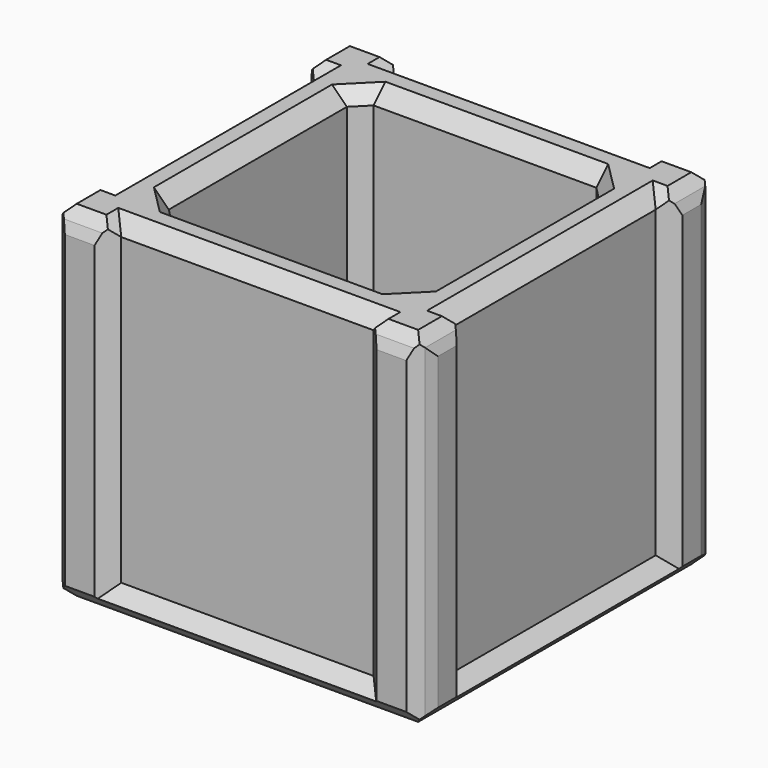
from build123d import *

# Parameters (mm, degrees)
F0_W          = 127
F0_H          = 127
F1_DEPTH      = 8.89
F2_W          = 86.36
F2_H          = 10.16
F2_W_2        = 10.16
F2_H_2        = 86.36
F3_DEPTH      = 101.6
F4_W          = 10.0171214116
F4_H          = 10.0171214116
F4_W_2        = 96.3771214116
F4_H_2        = 96.3771214116
F4_W_3        = 86.36
F4_H_3        = 86.36
F5_DEPTH      = 7.62
F6_W          = 86.36
F6_H          = 5.08
F9_W          = 5.08
F9_H          = 86.36
F7_W          = 5.08
F7_H          = 86.36
F8_W          = 86.36
F8_H          = 5.08
F10_DEPTH     = 109.22
F11_SIZE      = 5.08
F12_T1_DEPTH  = 139.1582991577
F12_T3_DEPTH  = 31.7862799398
F12_T5_DEPTH  = 153.1282991577
F12_T7_DEPTH  = 117.2041495789
F12_T9_DEPTH  = 86.36
F12_T11_DEPTH = 31.7862799398
F12_T17_DEPTH = 130.2682991577
F12_T22_DEPTH = 99.4241495789
F12_T29_DEPTH = 99.4241495789
F12_T33_DEPTH = 130.2682991577
F12_T41_DEPTH = 130.2682991577
F12_T46_DEPTH = 99.4241495789
F12_T53_DEPTH = 99.4241495789
F12_T57_DEPTH = 130.2682991577
F13_T1_DEPTH  = 124.4962799399
F13_T3_DEPTH  = 142.9682991577
F13_T5_DEPTH  = 26.7062799397
F13_T7_DEPTH  = 117.2041495789
F13_T9_DEPTH  = 86.36
F13_T11_DEPTH = 26.7062799398
F13_T17_DEPTH = 130.2682991577
F13_T22_DEPTH = 99.4241495789
F13_T29_DEPTH = 99.4241495789
F13_T33_DEPTH = 130.2682991577
F13_T41_DEPTH = 130.2682991577
F13_T46_DEPTH = 99.4241495789
F13_T53_DEPTH = 99.4241495789
F13_T57_DEPTH = 130.2682991577


# Not quite as in the source:
# - a fillet or chamfer that OpenCascade refuses, or shapes differently, is made with other operations: its cross-section is extruded or revolved along the edge and cut away or added


with BuildPart() as f1:
    # F0 (on Top) → F1 (new body)
    with BuildSketch(Plane.XY):
        with Locations((3.7135761231, -7.4630701935)):
            Rectangle(F0_W, F0_H)
    extrude(amount=F1_DEPTH)

    # F2 (on face) → F3 (join)
    with BuildSketch(Plane.XY.offset(8.89)):
        Polygon((-59.7864238769, 56.0369298065), (-59.7864238769, 35.7169298065), (-49.6264238769, 35.7169298065), (-39.4664238769, 35.7169298065), (-39.4664238769, 45.8769298065), (-39.4664238769, 56.0369298065), align=None)
        with Locations((3.7135761231, 40.7969298065)):
            Rectangle(F2_W, F2_H)
        Polygon((46.8935761231, 45.8769298065), (46.8935761231, 35.7169298065), (57.0535761231, 35.7169298065), (67.2135761231, 35.7169298065), (67.2135761231, 56.0369298065), (46.8935761231, 56.0369298065), align=None)
        with Locations((51.9735761231, -7.4630701935)):
            Rectangle(F2_W_2, F2_H_2)
        with Locations((-44.5464238769, -7.4630701935)):
            Rectangle(F2_W_2, F2_H_2)
        Polygon((-59.7864238769, -50.6430701935), (-59.7864238769, -70.9630701935), (-39.4664238769, -70.9630701935), (-39.4664238769, -60.8030701935), (-39.4664238769, -50.6430701935), (-49.6264238769, -50.6430701935), align=None)
        Polygon((46.8935761231, -60.8030701935), (46.8935761231, -70.9630701935), (67.2135761231, -70.9630701935), (67.2135761231, -50.6430701935), (57.0535761231, -50.6430701935), (46.8935761231, -50.6430701935), align=None)
        with Locations((3.7135761231, -55.7230701935)):
            Rectangle(F2_W, F2_H)
    extrude(amount=F3_DEPTH)

    # F4 (on face) → F5 (join)
    with BuildSketch(Plane.XY.offset(110.49)):
        Polygon((-39.4664238769, 56.0369298065), (-59.7864238769, 56.0369298065), (-59.7864238769, 35.7169298065), (-49.6264238769, 35.7169298065), (-49.6264238769, -50.6430701935), (-59.7864238769, -50.6430701935), (-59.7864238769, -70.9630701935), (-39.4664238769, -70.9630701935), (-39.4664238769, -60.8030701935), (46.8935761231, -60.8030701935), (46.8935761231, -70.9630701935), (67.2135761231, -70.9630701935), (67.2135761231, -50.6430701935), (57.0535761231, -50.6430701935), (57.0535761231, 35.7169298065), (67.2135761231, 35.7169298065), (67.2135761231, 56.0369298065), (46.8935761231, 56.0369298065), (46.8935761231, 45.8769298065), (-39.4664238769, 45.8769298065), align=None)
        with Locations((-49.6264238769, -60.8030701935)):
            Rectangle(F4_W, F4_H, mode=Mode.SUBTRACT)
        with Locations((57.0535761231, -60.8030701935)):
            Rectangle(F4_W, F4_H, mode=Mode.SUBTRACT)
        with Locations((-49.6264238769, 45.8769298065)):
            Rectangle(F4_W, F4_H, mode=Mode.SUBTRACT)
        with Locations((3.7135761231, -7.4630701935)):
            Rectangle(F4_W_2, F4_H_2, mode=Mode.SUBTRACT)
        with Locations((57.0535761231, 45.8769298065)):
            Rectangle(F4_W, F4_H, mode=Mode.SUBTRACT)
        with Locations((3.7135761231, -7.4630701935)):
            Rectangle(F4_W_2, F4_H_2)
        with Locations((3.7135761231, -7.4630701935)):
            Rectangle(F4_W_3, F4_H_3, mode=Mode.SUBTRACT)
        with Locations((-49.6264238769, 45.8769298065)):
            Rectangle(F4_W, F4_H)
        with Locations((57.0535761231, 45.8769298065)):
            Rectangle(F4_W, F4_H)
        with Locations((-49.6264238769, -60.8030701935)):
            Rectangle(F4_W, F4_H)
        with Locations((57.0535761231, -60.8030701935)):
            Rectangle(F4_W, F4_H)
    extrude(amount=F5_DEPTH)

    # F6 (on face) + F9 (on face) + F7 (on face) + F8 (on face) → F10 (join)
    with BuildSketch(Plane.XY.offset(8.89)):
        with Locations((3.7135761231, 48.4169298065)):
            Rectangle(F6_W, F6_H)
    with BuildSketch(Plane.XY.offset(8.89)):
        with Locations((-52.1664238769, -7.4630701935)):
            Rectangle(F9_W, F9_H)
    with BuildSketch(Plane.XY.offset(8.89)):
        with Locations((59.5935761231, -7.4630701935)):
            Rectangle(F7_W, F7_H)
    with BuildSketch(Plane.XY.offset(8.89)):
        with Locations((3.7135761231, -63.3430701935)):
            Rectangle(F8_W, F8_H)
    extrude(amount=F10_DEPTH)

    # F11
    f11_edges = [f1.edges().sort_by_distance(p)[0] for p in [
        (3.713576, -50.64307, 118.11),
        (-39.466424, -7.46307, 118.11),
        (3.713576, 35.71693, 118.11),
        (46.893576, -7.46307, 118.11),
        (67.213576, 45.87693, 118.11),
        (57.053576, 56.03693, 118.11),
        (46.893576, 53.49693, 118.11),
        (3.713576, 50.95693, 118.11),
        (-39.466424, 53.49693, 118.11),
        (-49.626424, 56.03693, 118.11),
        (-59.786424, 45.87693, 118.11),
        (-57.246424, 35.71693, 118.11),
        (-54.706424, -7.46307, 118.11),
        (-57.246424, -50.64307, 118.11),
        (-59.786424, -60.80307, 118.11),
        (-49.626424, -70.96307, 118.11),
        (-39.466424, -68.42307, 118.11),
        (3.713576, -65.88307, 118.11),
        (46.893576, -68.42307, 118.11),
        (57.053576, -70.96307, 118.11),
        (67.213576, -60.80307, 118.11),
        (64.673576, -50.64307, 118.11),
        (62.133576, -7.46307, 118.11),
        (64.673576, 35.71693, 118.11),
        (-39.466424, 35.71693, 63.5),
        (-39.466424, -7.46307, 8.89),
        (-39.466424, -50.64307, 63.5),
        (46.893576, 35.71693, 63.5),
        (3.713576, 35.71693, 8.89),
        (46.893576, -50.64307, 63.5),
        (46.893576, -7.46307, 8.89),
        (3.713576, -50.64307, 8.89),
    ]]
    chamfer(f11_edges, length=F11_SIZE)

    # F12: chamfer of 5.08 on 16 edges, made by hand

    # F12_s2 → F12_t1 (cut)
    with BuildSketch(Plane.XY.offset(-13.0641495789)):
        Polygon((67.2135761231, 50.9569298065), (62.1335761231, 56.0369298065), (67.2135761231, 56.0369298065), align=None)
        Polygon((-59.7864238769, 50.9569298065), (-54.7064238769, 56.0369298065), (-59.7864238769, 56.0369298065), align=None)
        Polygon((-54.7064238769, -70.9630701935), (-59.7864238769, -65.8830701935), (-59.7864238769, -70.9630701935), align=None)
        Polygon((62.1335761231, -70.9630701935), (67.2135761231, -65.8830701935), (67.2135761231, -70.9630701935), align=None)
    extrude(amount=F12_T1_DEPTH, mode=Mode.SUBTRACT)

    # F12_s4 → F12_t3 (cut)
    with BuildSketch(Plane.YZ.offset(41.1604361532)):
        Polygon((56.0369298065, 110.9257951031), (54.5490322549, 114.5178975516), (56.0369298065, 113.03), align=None)
        Polygon((-70.9630701935, 110.9257951031), (-69.4751726419, 114.5178975516), (-70.9630701935, 113.03), align=None)
    extrude(amount=F12_T3_DEPTH, mode=Mode.SUBTRACT)

    # F12_s6 → F12_t5 (cut)
    with BuildSketch(Plane.YZ.offset(-72.8505734557)):
        Polygon((50.9569298065, 0), (56.0369298065, 5.08), (56.0369298065, 0), align=None)
        Polygon((-70.9630701935, 5.08), (-65.8830701935, 0), (-70.9630701935, 0), align=None)
    extrude(amount=F12_T5_DEPTH, mode=Mode.SUBTRACT)

    # F12_s8 → F12_t7 (cut)
    with BuildSketch(Plane.XY.offset(8.89)):
        Polygon((51.9735761231, 56.0369298065), (46.8935761231, 50.9569298065), (46.8935761231, 56.0369298065), align=None)
        Polygon((-44.5464238769, 56.0369298065), (-39.4664238769, 50.9569298065), (-39.4664238769, 56.0369298065), align=None)
        Polygon((-44.5464238769, -70.9630701935), (-39.4664238769, -65.8830701935), (-39.4664238769, -70.9630701935), align=None)
        Polygon((51.9735761231, -70.9630701935), (46.8935761231, -65.8830701935), (46.8935761231, -70.9630701935), align=None)
    extrude(amount=F12_T7_DEPTH, mode=Mode.SUBTRACT)

    # F12_s10 → F12_t9 (cut)
    with BuildSketch(Plane.YZ.offset(-39.4664238769)):
        Polygon((56.0369298065, 3.81), (50.9569298065, 8.89), (56.0369298065, 8.89), align=None)
        Polygon((-70.9630701935, 3.81), (-65.8830701935, 8.89), (-70.9630701935, 8.89), align=None)
    extrude(amount=F12_T9_DEPTH, mode=Mode.SUBTRACT)

    # F12_s12 → F12_t11 (cut)
    with BuildSketch(Plane.YZ.offset(-65.5195638468)):
        Polygon((56.0369298065, 110.9257951031), (54.5490322549, 114.5178975516), (56.0369298065, 113.03), align=None)
        Polygon((-70.9630701935, 110.9257951031), (-69.4751726419, 114.5178975516), (-70.9630701935, 113.03), align=None)
    extrude(amount=F12_T11_DEPTH, mode=Mode.SUBTRACT)


with BuildPart() as f12_tool15:
    # F12_s16 → F12_t17 (new body)
    with BuildSketch(Plane.XY.offset(-4.1741495789)):
        Polygon((51.9735761231, 56.0369298065), (46.8935761231, 50.9569298065), (46.8935761231, 56.0369298065), align=None)
    extrude(amount=F12_T17_DEPTH)

    split(bisect_by=Plane.XY, keep=Keep.TOP)

    split(bisect_by=Plane.XY.offset(8.89), keep=Keep.BOTTOM)


with BuildPart() as f12_tool20:
    # F12_s21 → F12_t22 (new body)
    with BuildSketch(Plane.YZ.offset(59.957725702)):
        Polygon((56.0369298065, 3.81), (50.9569298065, 8.89), (56.0369298065, 8.89), align=None)
    extrude(amount=-F12_T22_DEPTH)

    split(bisect_by=Plane.YZ.offset(46.8935761231), keep=Keep.TOP)


with BuildPart() as f12_tool15_1:
    add(f12_tool15.part)

    # F12_t24: intersect F12_tool20
    add(f12_tool20.part, mode=Mode.INTERSECT)


with BuildPart() as f1_1:
    add(f1.part)

    # F12_t13: cut F12_tool15
    add(f12_tool15_1.part, mode=Mode.SUBTRACT)


with BuildPart() as f12_tool27:
    # F12_s28 → F12_t29 (new body)
    with BuildSketch(Plane.YZ.offset(46.8935761231)):
        Polygon((56.0369298065, 3.81), (50.9569298065, 8.89), (56.0369298065, 8.89), align=None)
    extrude(amount=-F12_T29_DEPTH)

    split(bisect_by=Plane.YZ.offset(-39.4664238769), keep=Keep.BOTTOM)


with BuildPart() as f12_tool31:
    # F12_s32 → F12_t33 (new body)
    with BuildSketch(Plane.XY.offset(126.0941495789)):
        Polygon((-44.5464238769, 56.0369298065), (-39.4664238769, 50.9569298065), (-39.4664238769, 56.0369298065), align=None)
    extrude(amount=-F12_T33_DEPTH)

    split(bisect_by=Plane.XY, keep=Keep.TOP)

    split(bisect_by=Plane.XY.offset(8.89), keep=Keep.BOTTOM)


with BuildPart() as f12_tool27_1:
    add(f12_tool27.part)

    # F12_t36: intersect F12_tool31
    add(f12_tool31.part, mode=Mode.INTERSECT)


with BuildPart() as f1_2:
    add(f1_1.part)

    # F12_t25: cut F12_tool27
    add(f12_tool27_1.part, mode=Mode.SUBTRACT)


with BuildPart() as f12_tool39:
    # F12_s40 → F12_t41 (new body)
    with BuildSketch(Plane.XY.offset(-4.1741495789)):
        Polygon((-44.5464238769, -70.9630701935), (-39.4664238769, -65.8830701935), (-39.4664238769, -70.9630701935), align=None)
    extrude(amount=F12_T41_DEPTH)

    split(bisect_by=Plane.XY, keep=Keep.TOP)

    split(bisect_by=Plane.XY.offset(8.89), keep=Keep.BOTTOM)


with BuildPart() as f12_tool44:
    # F12_s45 → F12_t46 (new body)
    with BuildSketch(Plane.YZ.offset(-52.5305734557)):
        Polygon((-70.9630701935, 3.81), (-65.8830701935, 8.89), (-70.9630701935, 8.89), align=None)
    extrude(amount=F12_T46_DEPTH)

    split(bisect_by=Plane.YZ.offset(-39.4664238769), keep=Keep.BOTTOM)


with BuildPart() as f12_tool39_1:
    add(f12_tool39.part)

    # F12_t48: intersect F12_tool44
    add(f12_tool44.part, mode=Mode.INTERSECT)


with BuildPart() as f1_3:
    add(f1_2.part)

    # F12_t37: cut F12_tool39
    add(f12_tool39_1.part, mode=Mode.SUBTRACT)


with BuildPart() as f12_tool51:
    # F12_s52 → F12_t53 (new body)
    with BuildSketch(Plane.YZ.offset(-39.4664238769)):
        Polygon((-70.9630701935, 3.81), (-65.8830701935, 8.89), (-70.9630701935, 8.89), align=None)
    extrude(amount=F12_T53_DEPTH)

    split(bisect_by=Plane.YZ.offset(46.8935761231), keep=Keep.TOP)


with BuildPart() as f12_tool55:
    # F12_s56 → F12_t57 (new body)
    with BuildSketch(Plane.XY.offset(126.0941495789)):
        Polygon((51.9735761231, -70.9630701935), (46.8935761231, -65.8830701935), (46.8935761231, -70.9630701935), align=None)
    extrude(amount=-F12_T57_DEPTH)

    split(bisect_by=Plane.XY, keep=Keep.TOP)

    split(bisect_by=Plane.XY.offset(8.89), keep=Keep.BOTTOM)


with BuildPart() as f12_tool51_1:
    add(f12_tool51.part)

    # F12_t60: intersect F12_tool55
    add(f12_tool55.part, mode=Mode.INTERSECT)


with BuildPart() as f1_4:
    add(f1_3.part)

    # F12_t49: cut F12_tool51
    add(f12_tool51_1.part, mode=Mode.SUBTRACT)

    # F13: chamfer of 5.08 on 16 edges, made by hand

    # F13_s2 → F13_t1 (cut)
    with BuildSketch(Plane.XY.offset(-5.7331399699)):
        Polygon((-59.7864238769, 48.8527249097), (-58.2985263253, 52.4448273581), (-59.7864238769, 50.9569298065), align=None)
        Polygon((-59.7864238769, -63.7788652967), (-58.2985263253, -67.3709677451), (-59.7864238769, -65.8830701935), align=None)
        Polygon((65.7256785715, -67.3709677451), (67.2135761231, -63.7788652966), (67.2135761231, -65.8830701935), align=None)
        Polygon((65.7256785715, 52.4448273581), (67.2135761231, 48.8527249096), (67.2135761231, 50.9569298065), align=None)
    extrude(amount=F13_T1_DEPTH, mode=Mode.SUBTRACT)

    # F13_s4 → F13_t3 (cut)
    with BuildSketch(Plane.XZ.offset(-64.0210793854)):
        Polygon((-59.7864238769, 5.08), (-54.7064238769, 0), (-59.7864238769, 0), align=None)
        Polygon((62.1335761231, 0), (67.2135761231, 5.08), (67.2135761231, 0), align=None)
    extrude(amount=F13_T3_DEPTH, mode=Mode.SUBTRACT)

    # F13_s6 → F13_t5 (cut)
    with BuildSketch(Plane.XZ.offset(44.9099302236)):
        Polygon((-58.2985263253, 114.5178975516), (-59.7864238769, 110.9257951031), (-59.7864238769, 113.03), align=None)
        Polygon((65.7256785715, 114.5178975516), (67.2135761231, 110.9257951031), (67.2135761231, 113.03), align=None)
    extrude(amount=F13_T5_DEPTH, mode=Mode.SUBTRACT)

    # F13_s8 → F13_t7 (cut)
    with BuildSketch(Plane.XY.offset(8.89)):
        Polygon((-59.7864238769, -55.7230701935), (-54.7064238769, -50.6430701935), (-59.7864238769, -50.6430701935), align=None)
        Polygon((-59.7864238769, 40.7969298065), (-54.7064238769, 35.7169298065), (-59.7864238769, 35.7169298065), align=None)
        Polygon((62.1335761231, 35.7169298065), (67.2135761231, 40.7969298065), (67.2135761231, 35.7169298065), align=None)
        Polygon((62.1335761231, -50.6430701935), (67.2135761231, -55.7230701935), (67.2135761231, -50.6430701935), align=None)
    extrude(amount=F13_T7_DEPTH, mode=Mode.SUBTRACT)

    # F13_s10 → F13_t9 (cut)
    with BuildSketch(Plane.XZ.offset(-35.7169298065)):
        Polygon((-59.7864238769, 3.81), (-54.7064238769, 8.89), (-59.7864238769, 8.89), align=None)
        Polygon((62.1335761231, 8.89), (67.2135761231, 3.81), (67.2135761231, 8.89), align=None)
    extrude(amount=F13_T9_DEPTH, mode=Mode.SUBTRACT)

    # F13_s12 → F13_t11 (cut)
    with BuildSketch(Plane.XZ.offset(-56.6900697764)):
        Polygon((-59.7864238769, 110.9257951031), (-58.2985263253, 114.5178975516), (-59.7864238769, 113.03), align=None)
        Polygon((65.7256785715, 114.5178975516), (67.2135761231, 110.9257951031), (67.2135761231, 113.03), align=None)
    extrude(amount=F13_T11_DEPTH, mode=Mode.SUBTRACT)


with BuildPart() as f13_tool15:
    # F13_s16 → F13_t17 (new body)
    with BuildSketch(Plane.XY.offset(126.0941495789)):
        Polygon((-59.7864238769, -55.7230701935), (-54.7064238769, -50.6430701935), (-59.7864238769, -50.6430701935), align=None)
    extrude(amount=-F13_T17_DEPTH)

    split(bisect_by=Plane.XY.offset(8.89), keep=Keep.BOTTOM)

    split(bisect_by=Plane.XY, keep=Keep.TOP)


with BuildPart() as f13_tool20:
    # F13_s21 → F13_t22 (new body)
    with BuildSketch(Plane.XZ.offset(-35.7169298065)):
        Polygon((-59.7864238769, 3.81), (-54.7064238769, 8.89), (-59.7864238769, 8.89), align=None)
    extrude(amount=F13_T22_DEPTH)

    split(bisect_by=Plane.XZ.offset(50.6430701935), keep=Keep.TOP)


with BuildPart() as f13_tool15_1:
    add(f13_tool15.part)

    # F13_t24: intersect F13_tool20
    add(f13_tool20.part, mode=Mode.INTERSECT)


with BuildPart() as f1_5:
    add(f1_4.part)

    # F13_t13: cut F13_tool15
    add(f13_tool15_1.part, mode=Mode.SUBTRACT)


with BuildPart() as f13_tool27:
    # F13_s28 → F13_t29 (new body)
    with BuildSketch(Plane.XZ.offset(-48.7810793854)):
        Polygon((-59.7864238769, 3.81), (-54.7064238769, 8.89), (-59.7864238769, 8.89), align=None)
    extrude(amount=F13_T29_DEPTH)

    split(bisect_by=Plane.XZ.offset(-35.7169298065), keep=Keep.BOTTOM)


with BuildPart() as f13_tool31:
    # F13_s32 → F13_t33 (new body)
    with BuildSketch(Plane.XY.offset(-4.1741495789)):
        Polygon((-59.7864238769, 40.7969298065), (-54.7064238769, 35.7169298065), (-59.7864238769, 35.7169298065), align=None)
    extrude(amount=F13_T33_DEPTH)

    split(bisect_by=Plane.XY.offset(8.89), keep=Keep.BOTTOM)

    split(bisect_by=Plane.XY, keep=Keep.TOP)


with BuildPart() as f13_tool27_1:
    add(f13_tool27.part)

    # F13_t36: intersect F13_tool31
    add(f13_tool31.part, mode=Mode.INTERSECT)


with BuildPart() as f1_6:
    add(f1_5.part)

    # F13_t25: cut F13_tool27
    add(f13_tool27_1.part, mode=Mode.SUBTRACT)


with BuildPart() as f13_tool39:
    # F13_s40 → F13_t41 (new body)
    with BuildSketch(Plane.XY.offset(126.0941495789)):
        Polygon((62.1335761231, 35.7169298065), (67.2135761231, 40.7969298065), (67.2135761231, 35.7169298065), align=None)
    extrude(amount=-F13_T41_DEPTH)

    split(bisect_by=Plane.XY, keep=Keep.TOP)

    split(bisect_by=Plane.XY.offset(8.89), keep=Keep.BOTTOM)


with BuildPart() as f13_tool44:
    # F13_s45 → F13_t46 (new body)
    with BuildSketch(Plane.XZ.offset(50.6430701935)):
        Polygon((62.1335761231, 8.89), (67.2135761231, 3.81), (67.2135761231, 8.89), align=None)
    extrude(amount=-F13_T46_DEPTH)

    split(bisect_by=Plane.XZ.offset(-35.7169298065), keep=Keep.BOTTOM)


with BuildPart() as f13_tool39_1:
    add(f13_tool39.part)

    # F13_t48: intersect F13_tool44
    add(f13_tool44.part, mode=Mode.INTERSECT)


with BuildPart() as f1_7:
    add(f1_6.part)

    # F13_t37: cut F13_tool39
    add(f13_tool39_1.part, mode=Mode.SUBTRACT)


with BuildPart() as f13_tool51:
    # F13_s52 → F13_t53 (new body)
    with BuildSketch(Plane.XZ.offset(63.7072197724)):
        Polygon((62.1335761231, 8.89), (67.2135761231, 3.81), (67.2135761231, 8.89), align=None)
    extrude(amount=-F13_T53_DEPTH)

    split(bisect_by=Plane.XZ.offset(50.6430701935), keep=Keep.TOP)


with BuildPart() as f13_tool55:
    # F13_s56 → F13_t57 (new body)
    with BuildSketch(Plane.XY.offset(-4.1741495789)):
        Polygon((62.1335761231, -50.6430701935), (67.2135761231, -55.7230701935), (67.2135761231, -50.6430701935), align=None)
    extrude(amount=F13_T57_DEPTH)

    split(bisect_by=Plane.XY, keep=Keep.TOP)

    split(bisect_by=Plane.XY.offset(8.89), keep=Keep.BOTTOM)


with BuildPart() as f13_tool51_1:
    add(f13_tool51.part)

    # F13_t60: intersect F13_tool55
    add(f13_tool55.part, mode=Mode.INTERSECT)


with BuildPart() as f1_8:
    add(f1_7.part)

    # F13_t49: cut F13_tool51
    add(f13_tool51_1.part, mode=Mode.SUBTRACT)


solid = f1_8.part
